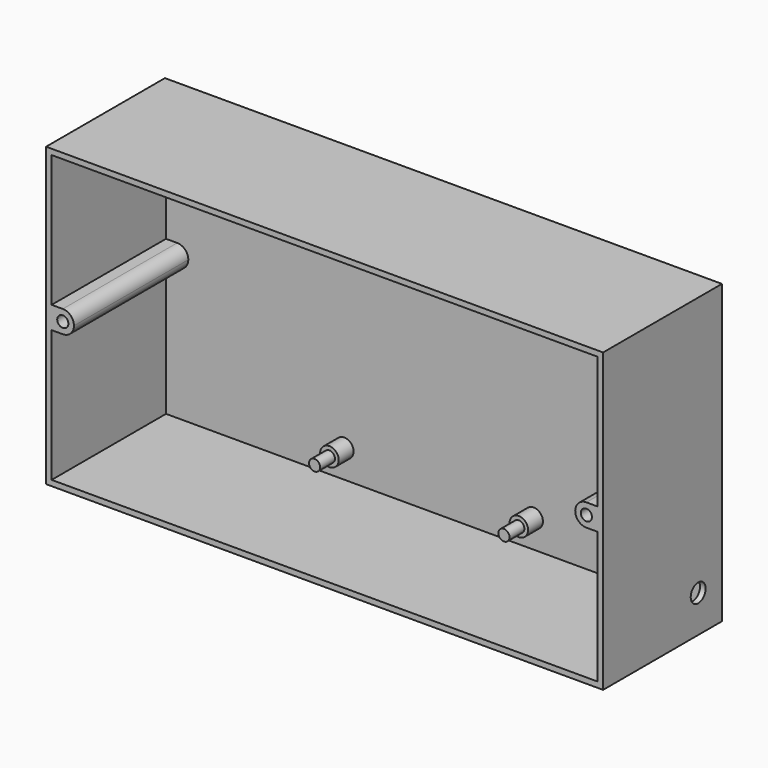
from build123d import *

# Parameters (mm, degrees)
F0_W      = 150
F0_H      = 80
F1_DEPTH  = 40
F2_W      = 147
F2_H      = 77
F3_DEPTH  = 38.5
F4_R      = 2.5
F5_DEPTH  = 5
F6_R      = 1.5
F7_R      = 1.5
F8_R      = 1.5
F9_R      = 1.5
F10_DEPTH = 5
F11_R     = 2.5
F12_DEPTH = 3
F13_W     = 6
F13_H     = 6
F14_DEPTH = 38.5
F15_R     = 1.5
F16_DEPTH = 35
F17_R     = 2.99999


# Not quite as in the source:
# - a fillet or chamfer is up to 0.001 mm smaller than in the source, because OpenCascade refuses the exact size


with BuildPart() as f1:
    # F0 (on Front) → F1 (new body)
    with BuildSketch(Plane.XZ):
        Rectangle(F0_W, F0_H)
    extrude(amount=F1_DEPTH)

    # F2 (on face) → F3 (cut)
    with BuildSketch(Plane.XZ.offset(40)):
        Rectangle(F2_W, F2_H)
    extrude(amount=-F3_DEPTH, mode=Mode.SUBTRACT)

    # F4 (on face) → F5 (join)
    with BuildSketch(Plane.XZ.offset(1.5)):
        with Locations((-25.5, 31)):
            Circle(F4_R)
        with Locations((-25.5, -31)):
            Circle(F4_R)
        with Locations((25.5, 31)):
            Circle(F4_R)
        with Locations((25.5, -31)):
            Circle(F4_R)
    extrude(amount=F5_DEPTH)

    # F6 (on face) + F7 (on face) + F8 (on face) + F9 (on face) → F10 (join)
    with BuildSketch(Plane.XZ.offset(6.5)):
        with Locations((-25.5, 31)):
            Circle(F6_R)
    with BuildSketch(Plane.XZ.offset(6.5)):
        with Locations((25.5, 31)):
            Circle(F7_R)
    with BuildSketch(Plane.XZ.offset(6.5)):
        with Locations((-25.5, -31)):
            Circle(F8_R)
    with BuildSketch(Plane.XZ.offset(6.5)):
        with Locations((25.5, -31)):
            Circle(F9_R)
    extrude(amount=F10_DEPTH)

    # F11 (on face) → F12 (cut)
    with BuildSketch(Plane.YZ.offset(75)):
        with Locations((-8, -30)):
            Circle(F11_R)
    extrude(amount=-F12_DEPTH, mode=Mode.SUBTRACT)

    # F13 (on face) → F14 (join)
    with BuildSketch(Plane.XZ.offset(1.5)):
        with Locations((-70.5, 0)):
            Rectangle(F13_W, F13_H)
        with Locations((70.5, 0)):
            Rectangle(F13_W, F13_H)
    extrude(amount=F14_DEPTH)

    # F15 (on face) → F16 (cut)
    with BuildSketch(Plane.XZ.offset(40)):
        with Locations((-70.5, 0)):
            Circle(F15_R)
        with Locations((70.5, 0)):
            Circle(F15_R)
    extrude(amount=-F16_DEPTH, mode=Mode.SUBTRACT)

    # F17 (radius 3 in the source; OpenCascade refuses exactly that, so slightly less here)
    f17_edges = [f1.edges().sort_by_distance(p)[0] for p in [
        (-67.5, -20.75, 3),
        (-67.5, -20.75, -3),
        (67.5, -20.75, -3),
        (67.5, -20.75, 3),
    ]]
    fillet(f17_edges, radius=F17_R)


solid = f1.part
